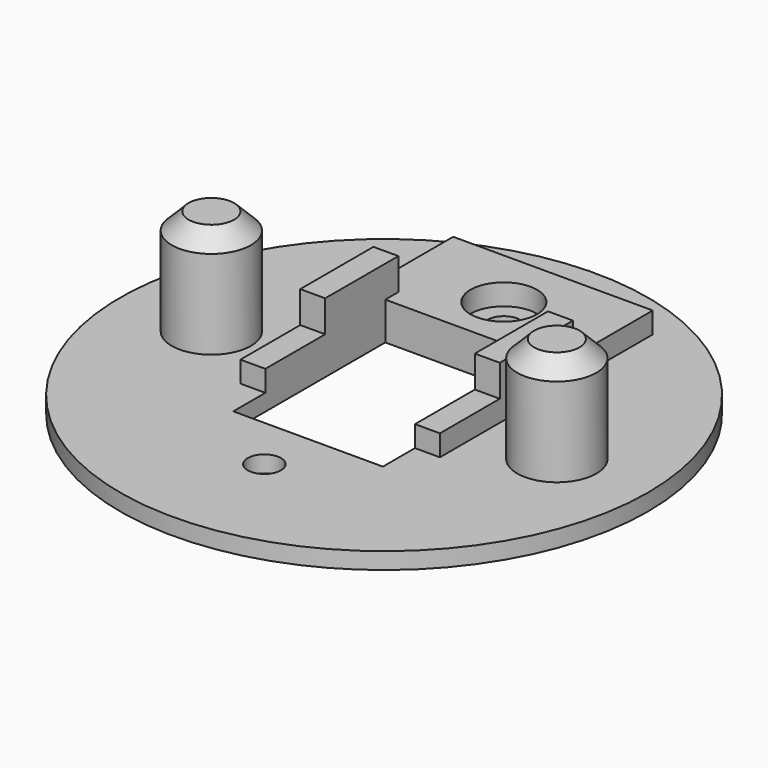
from build123d import *

# Parameters (mm, degrees)
F0_R     = 15.875
F0_R_2   = 1
F0_W     = 9
F0_H     = 11.43
F1_DEPTH = 1
F2_R     = 2
F3_DEPTH = 1.27
F4_W     = 1.5
F4_H     = 5.5
F5_DEPTH = 1.905
F6_R     = 2.38125
F7_DEPTH = 6.35
F8_SIZE  = 1.016


# Not quite as in the source:
# - a pattern or mirror of a feature is missing from the dataset's text; its kind, count and spacing are read off the source's solid


with BuildPart() as f1:
    # F0 (on Top) → F1 (new body)
    with BuildSketch(Plane.XY):
        Circle(F0_R)
        with Locations((0, -9)):
            Circle(F0_R_2, mode=Mode.SUBTRACT)
        Rectangle(F0_W, F0_H, mode=Mode.SUBTRACT)
        with Locations((0, 9)):
            Circle(F0_R_2, mode=Mode.SUBTRACT)
    extrude(amount=F1_DEPTH)

    # F2 (on face) → F3 (join)
    with BuildSketch(Plane.XY.offset(1)):
        Polygon((6, 12.6974700204), (-6, 12.6974700204), (-6, -3.3025299796), (-4.5, -3.3025299796), (-4.5, 5.715), (4.5, 5.715), (4.5, -3.3025299796), (6, -3.3025299796), align=None)
        with Locations((0, 9)):
            Circle(F2_R, mode=Mode.SUBTRACT)
    extrude(amount=F3_DEPTH)

    # F4 (on face) → F5 (join)
    with BuildSketch(Plane.XY.offset(2.27)):
        with Locations((-5.25, 3.9474700204)):
            Rectangle(F4_W, F4_H)
    f5 = extrude(amount=F5_DEPTH)

    # F5_copies: F5 across plane
    add(f5.mirror(Plane(origin=(0, 0, 0), x_dir=(0, 0, 1), z_dir=(1, 0, 0))))

    # F6 (on face) → F7 (join)
    with BuildSketch(Plane.XY.offset(1)):
        with Locations((10.3898039088, 0)):
            Circle(F6_R)
        with Locations((-10.3898039088, 0)):
            Circle(F6_R)
    extrude(amount=F7_DEPTH)

    # F8
    f8_edges = [f1.edges().sort_by_distance(p)[0] for p in [
        (-12.771054, 0, 7.35),
        (8.008554, 0, 7.35),
    ]]
    chamfer(f8_edges, length=F8_SIZE)


solid = f1.part
